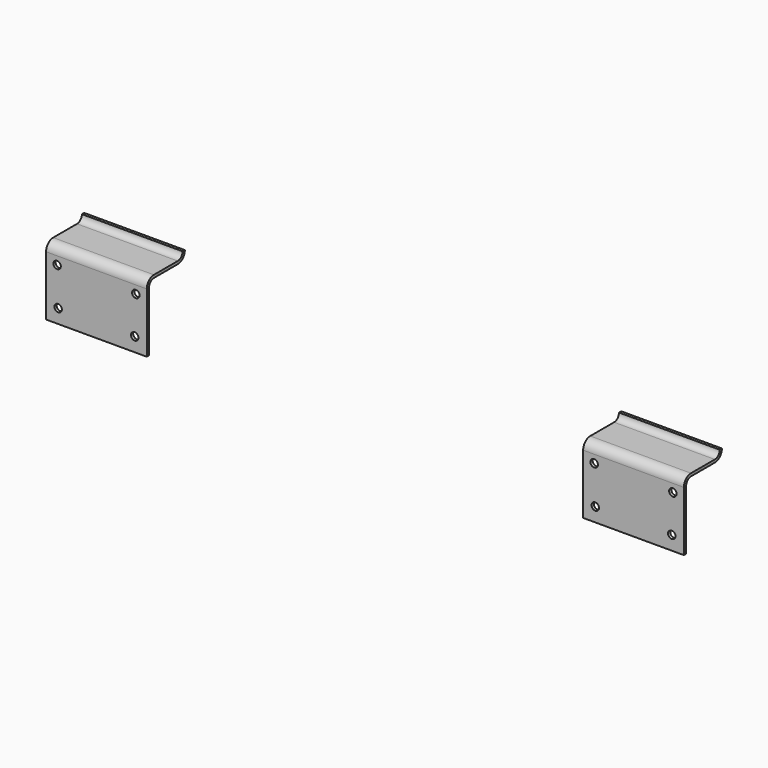
from build123d import *

# Parameters (mm, degrees)
F1_W     = 171.45
F1_H     = 4.7625
F3_R     = 6.35
F4_DEPTH = 80.9635


with BuildPart() as f2:
    # F2: sweep along a path in F0
    with BuildLine(Plane.YZ) as f2_path:
        Line((0, 0), (0, 101.6))
        ThreePointArc((0, 101.6), (3.7197438789, 110.5802561211), (12.7, 114.3))
        Line((12.7, 114.3), (63.5, 114.3))
        ThreePointArc((63.5, 114.3), (72.4802561211, 118.0197438789), (76.2, 127))
    # F1 (on Top) → F2 (sweep)
    with BuildSketch(Plane.XY):
        Rectangle(F1_W, F1_H)
    sweep(path=f2_path.line)

    # F3 (on face) → F4 (cut, through all)
    with BuildSketch(Plane.XZ.offset(2.38125)):
        with Locations((-67.0052, 87.9475)):
            Circle(F3_R)
        with Locations((67.0052, 87.9475)):
            Circle(F3_R)
        with Locations((-65.1383, 23.8125)):
            Circle(F3_R)
        with Locations((65.1383, 23.8125)):
            Circle(F3_R)
    extrude(amount=-F4_DEPTH, mode=Mode.SUBTRACT)


with BuildPart() as f5_1:
    # F5: copy of F2
    add(f2.part.moved(Location((914.4, 0, 0))))


solid = Compound([f2.part, f5_1.part])
